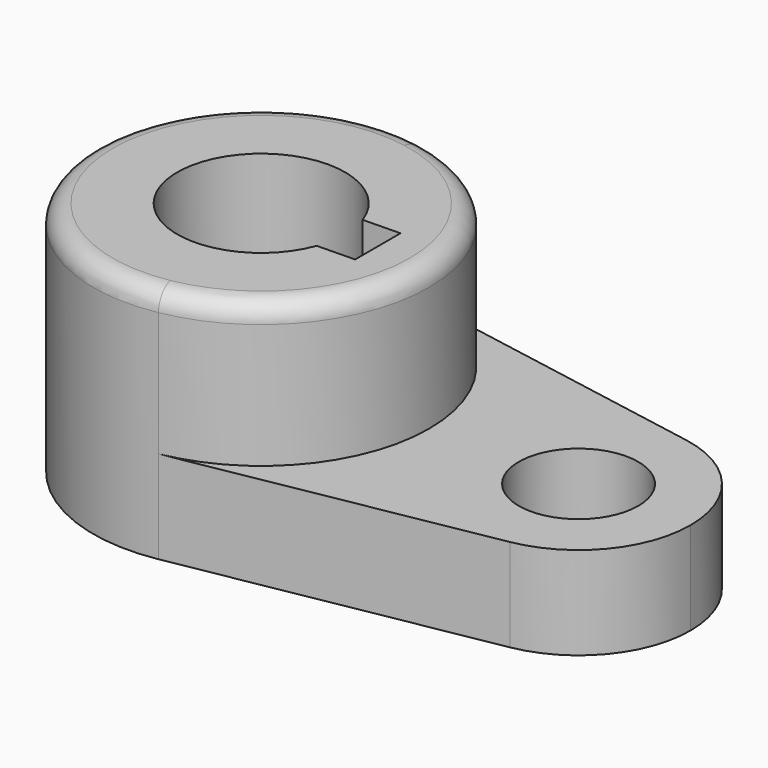
from build123d import *

# Parameters (mm, degrees)
F1_DEPTH = 40.2336
F0_R     = 10.16
F2_DEPTH = 15.7734
F3_R     = 3.302


# Not quite as in the source:
# - a feature names something its author has since deleted; it is built from what else it names


with BuildPart() as f1:
    # F0 (on Top) → F1 (new body)
    with BuildSketch(Plane.XY):
        with BuildLine():
            ThreePointArc((5.0426470588, -28.1265414802), (21.9160245563, -18.3362616868), (28.575, 0))
            ThreePointArc((28.575, 0), (21.9160245563, 18.3362616868), (5.0426470588, 28.1265414802))
            ThreePointArc((5.0426470588, 28.1265414802), (-28.575, 0), (5.0426470588, -28.1265414802))
        make_face()
        with BuildLine():
            ThreePointArc((13.4021500625, -4.9512654901), (-14.2868886671, 0.1321683185), (13.4914569997, 4.702472145))
            Line((13.4914569997, 4.702472145), (19.8402553797, 4.826))
            Line((19.8402553797, 4.826), (19.8402553797, -4.826))
            Line((19.8402553797, -4.826), (13.4021500625, -4.9512654901))
        make_face(mode=Mode.SUBTRACT)
    extrude(amount=F1_DEPTH)

    # F0 (on Top) → F2 (join)
    with BuildSketch(Plane.XY):
        with BuildLine():
            ThreePointArc((5.0426470588, 28.1265414802), (21.9160245563, 18.3362616868), (28.575, 0))
            ThreePointArc((28.575, 0), (21.9160245563, -18.3362616868), (5.0426470588, -28.1265414802))
            Line((5.0426470588, -28.1265414802), (57.3367647059, -18.7510276535))
            ThreePointArc((57.3367647059, -18.7510276535), (34.925, 0), (57.3367647059, 18.7510276535))
            Line((57.3367647059, 18.7510276535), (5.0426470588, 28.1265414802))
        make_face()
        with BuildLine():
            ThreePointArc((73.025, 0), (68.5856830375, 12.2241744579), (57.3367647059, 18.7510276535))
            ThreePointArc((57.3367647059, 18.7510276535), (34.925, 0), (57.3367647059, -18.7510276535))
            ThreePointArc((57.3367647059, -18.7510276535), (68.5856830375, -12.2241744579), (73.025, 0))
        make_face()
        with Locations((53.975, 0)):
            Circle(F0_R, mode=Mode.SUBTRACT)
    extrude(amount=F2_DEPTH)

    # F3
    f3_edges = [f1.edges().sort_by_distance(p)[0] for p in [
        (-5.042647, 28.126541, 40.2336),
    ]]
    fillet(f3_edges, radius=F3_R)


solid = f1.part
